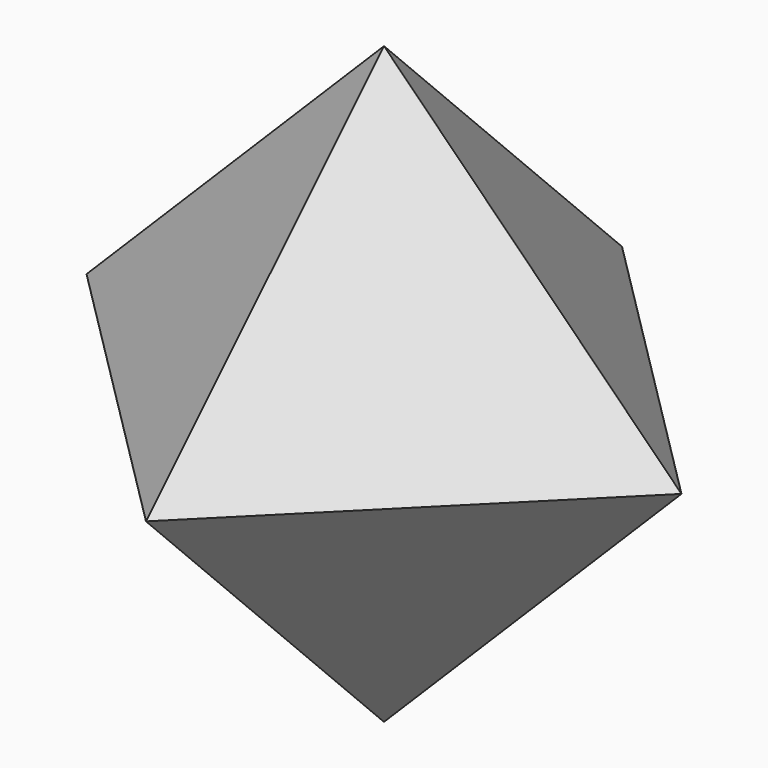
from build123d import *

# Parameters (mm, degrees)
F0_W     = 50.8
F0_H     = 50.8
F1_DEPTH = 25.4
F2_SIZE  = 25.39999


# Not quite as in the source:
# - a fillet or chamfer is up to 0.001 mm smaller than in the source, because OpenCascade refuses the exact size


with BuildPart() as f1:
    # F0 (on Front) → F1 (new body, symmetric)
    with BuildSketch(Plane.XZ):
        Rectangle(F0_W, F0_H)
    extrude(amount=F1_DEPTH, both=True)

    # F2 (size 25.4 in the source; OpenCascade refuses exactly that, so slightly less here)
    f2_edges = [f1.edges().sort_by_distance(p)[0] for p in [
        (0, 25.4, -25.4),
        (25.4, 0, -25.4),
        (0, -25.4, -25.4),
        (-25.4, 0, -25.4),
        (25.4, 25.4, 0),
        (0, 25.4, 25.4),
        (-25.4, 25.4, 0),
        (25.4, 0, 25.4),
        (25.4, -25.4, 0),
        (0, -25.4, 25.4),
        (-25.4, -25.4, 0),
        (-25.4, 0, 25.4),
    ]]
    chamfer(f2_edges, length=F2_SIZE)


solid = f1.part
